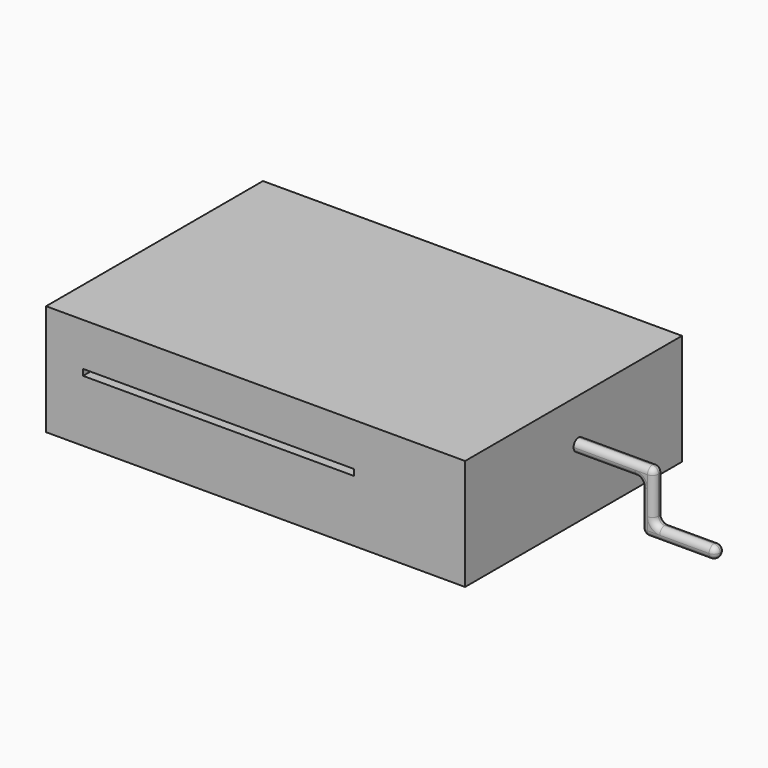
from build123d import *

# Parameters (mm, degrees)
F1_DEPTH      = 28.575
F2_W          = 69.85
F2_H          = 1.5875
F3_DEPTH      = 69.85
F6_DEPTH      = 1.5875
F6_DEPTH_BACK = 1.5875
F7_R          = 1.58749


# Not quite as in the source:
# - a fillet or chamfer is up to 0.001 mm smaller than in the source, because OpenCascade refuses the exact size


with BuildPart() as f1:
    # F0 (on Top) → F1 (new body)
    with BuildSketch(Plane.XY):
        Polygon((53.975, -34.925), (53.975, 0), (53.975, 34.925), (-53.975, 34.925), (-53.975, -34.925), align=None)
    extrude(amount=F1_DEPTH)

    # F2 (on face) → F3 (cut, through all)
    with BuildSketch(Plane.XZ.offset(34.925)):
        with Locations((-9.525, 16.66875)):
            Rectangle(F2_W, F2_H)
    extrude(amount=-F3_DEPTH, mode=Mode.SUBTRACT)

    # F5 (on offset) → F6 (join, two sides)
    with BuildSketch(Plane.XZ.offset(-1.5875)) as f6_sk:
        Polygon((53.975, 19.05), (53.975, 15.875), (71.4375, 15.875), (71.4375, 3.175), (90.4875, 3.175), (90.4875, 6.35), (74.6125, 6.35), (74.6125, 19.05), align=None)
    extrude(amount=F6_DEPTH)
    extrude(f6_sk.sketch, amount=-F6_DEPTH_BACK)

    # F7 (radius 1.5875 in the source; OpenCascade refuses exactly that, so slightly less here)
    f7_edges = [f1.edges().sort_by_distance(p)[0] for p in [
        (64.29375, 0, 19.05),
        (74.6125, 3.175, 12.7),
        (74.6125, 0, 12.7),
        (74.6125, 1.5875, 19.05),
        (74.6125, 1.5875, 6.35),
        (71.4375, 0, 9.525),
        (62.70625, 0, 15.875),
        (64.29375, 3.175, 19.05),
        (82.55, 3.175, 6.35),
        (82.55, 0, 6.35),
        (80.9625, 0, 3.175),
        (90.4875, 1.5875, 3.175),
        (90.4875, 0, 4.7625),
        (90.4875, 1.5875, 6.35),
        (90.4875, 3.175, 4.7625),
        (62.70625, 3.175, 15.875),
        (71.4375, 1.5875, 3.175),
        (80.9625, 3.175, 3.175),
        (71.4375, 3.175, 9.525),
        (71.4375, 1.5875, 15.875),
    ]]
    fillet(f7_edges, radius=F7_R)


solid = f1.part
